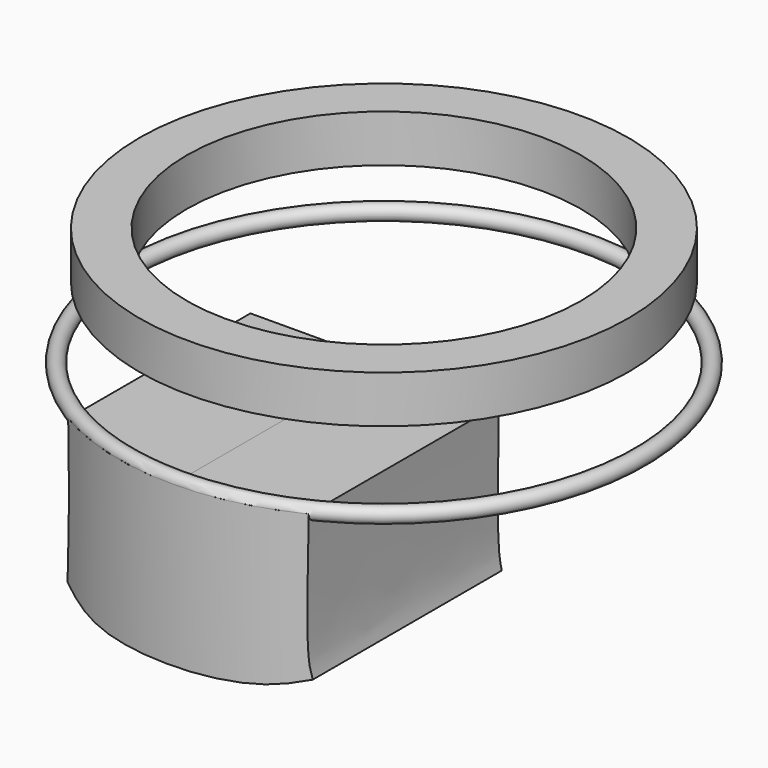
from build123d import *

# Parameters (mm, degrees)
F1_R      = 0.5
F4_DEPTH  = 20
F5_W      = 10
F5_H      = 10.4441631917
F7_W      = 15.5
F7_H      = 3
F9_R      = 12.5
F10_DEPTH = 17.6481520487


with BuildPart() as f2:
    # F1 (on face) → F2 (revolve)
    with BuildSketch(Plane.XZ):
        with Locations((-16.2385423089, -12.5)):
            Circle(F1_R)
    revolve(axis=Axis((0, 0, -13.5), (0, 0, -1)))

    # F3 (on Front) → F4 (join)
    with BuildSketch(Plane.XZ):
        with BuildLine():
            Line((0, -12.4902276899), (-8.4660975263, -12.515693903))
            add(Edge.make_bspline(
                [(-8.4660975263, -12.515693903), (-8.4193508372, -14.191675073), (-8.329257132, -17.4217509736), (-8.4736987191, -20.3036586232), (-8.5431942716, -21.6902382672)],
                knots=[0, 0, 0, 0, 0.5188674265, 1, 1, 1, 1], degree=3))
            add(Edge.make_bspline(
                [(-8.5431942716, -21.6902382672), (-7.8688632415, -21.9706217142), (-6.2298852231, -22.652100522), (-1.5468896764, -22.6523203072), (4.7965653474, -22.6082263247), (6.7166952245, -21.949377428), (7.471922785, -21.6902382672)],
                knots=[0, 0, 0, 0, 0.1935734996, 0.4704851129, 0.7917306318, 1, 1, 1, 1], degree=3))
            add(Edge.make_bspline(
                [(7.2885542177, -12.4683035538), (7.2738022544, -13.4565242356), (7.2413210861, -15.632408325), (7.1902968982, -20.465056858), (7.4018706428, -21.3854843849), (7.471922785, -21.6902382672)],
                knots=[0, 0, 0, 0, 0.3575627357, 0.7872887927, 1, 1, 1, 1], degree=3))
            Line((7.2885542177, -12.4683035538), (0, -12.4902276899))
        make_face()
    extrude(amount=F4_DEPTH)

    # F5 (on Front) → F6 (revolve, cut)
    with BuildSketch(Plane.XZ):
        with Locations((-21.739, -17.6152454027)):
            Rectangle(F5_W, F5_H)
    revolve(axis=Axis((0, 0, -16.7107414454), (0, 0, -1)), mode=Mode.SUBTRACT)


with BuildPart() as f8:
    # F7 (on Front) → F8 (revolve)
    with BuildSketch(Plane.XZ):
        with Locations((-7.75, -6.5)):
            Rectangle(F7_W, F7_H)
    revolve(axis=Axis((0, 0, -6.5), (0, 0, 1)))

    # F9 (on face) → F10 (cut, through all)
    with BuildSketch(Plane.XY.offset(-5)):
        Circle(F9_R)
    extrude(amount=-F10_DEPTH, mode=Mode.SUBTRACT)


solid = Compound([f2.part, f8.part])
